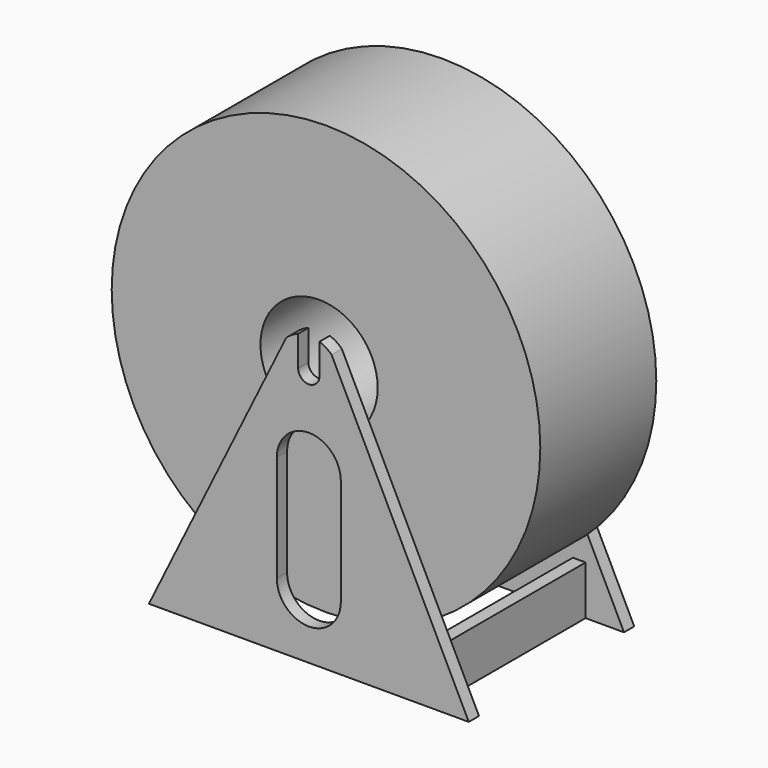
from build123d import *

# Parameters (mm, degrees)
F0_R      = 100.5
F0_R_2    = 27.5
F1_DEPTH  = 34
F3_DEPTH  = 6
F4_W      = 150
F4_H      = 6
F5_DEPTH  = 85
F9_DEPTH  = 122
F12_W     = 85
F12_H     = 36.2278819084
F13_DEPTH = 172
F14_W     = 6
F14_H     = 23
F15_DEPTH = 85


# Not quite as in the source:
# - a feature of the source that left no trace in its solid (it failed there, or was rolled back) is left out
# - a feature names something its author has since deleted; it is built from what else it names


with BuildPart() as f1:
    # F0 (on Front) → F1 (new body, symmetric)
    with BuildSketch(Plane.XZ):
        with Locations((3.2501332462, 0)):
            Circle(F0_R)
        Circle(F0_R_2, mode=Mode.SUBTRACT)
    extrude(amount=F1_DEPTH, both=True)


with BuildPart() as f3:
    # F2 (on face) → F3 (new body)
    with BuildSketch(Plane.XZ.offset(34)):
        with BuildLine():
            ThreePointArc((82.7773839779, -61.4464514114), (0.9255990786, -100.4731135225), (-79.0337407783, -57.7028082117))
            Line((-79.0337407783, -57.7028082117), (-141.3309325666, -120))
            Line((-141.3309325666, -120), (141.3309325666, -120))
            Line((141.3309325666, -120), (82.7773839779, -61.4464514114))
        make_face()
        with BuildLine():
            ThreePointArc((26.9250120629, -5.5940794963), (0, -27.5), (-26.9250120629, -5.5940794963))
            Line((-26.9250120629, -5.5940794963), (-79.0337407783, -57.7028082117))
            ThreePointArc((-79.0337407783, -57.7028082117), (0.9255990786, -100.4731135225), (82.7773839779, -61.4464514114))
            Line((82.7773839779, -61.4464514114), (26.9250120629, -5.5940794963))
        make_face()
        with BuildLine():
            Line((-5, 0), (-5, 14.2304020351))
            ThreePointArc((-5, 14.2304020351), (-8.0329882483, 12.7661835285), (-10.6654662833, 10.6654662833))
            Line((-10.6654662833, 10.6654662833), (-26.9250120629, -5.5940794963))
            ThreePointArc((-26.9250120629, -5.5940794963), (0, -27.5), (26.9250120629, -5.5940794963))
            Line((26.9250120629, -5.5940794963), (10.6654662833, 10.6654662833))
            ThreePointArc((10.6654662833, 10.6654662833), (8.0329882483, 12.7661835285), (5, 14.2304020351))
            Line((5, 14.2304020351), (5, 0))
            ThreePointArc((5, 0), (0, -5), (-5, 0))
        make_face()
    extrude(amount=F3_DEPTH)

    # F4 (on face) → F5 (join)
    with BuildSketch(Plane(origin=(0, -34, 0), x_dir=(-1, 0, 0), z_dir=(0, 1, 0))):
        with Locations((0, -117)):
            Rectangle(F4_W, F4_H)
    extrude(amount=F5_DEPTH)

    # F7: F3 across plane


with BuildPart() as f3_1:
    add(f3.part)
    add(f3.part.mirror(Plane(origin=(0, 8.5, -94.3962931942), x_dir=(-1, 0, 0), z_dir=(0, 1, 0))))

    # F8 (on face) → F9 (cut)
    with BuildSketch(Plane.XZ.offset(40)):
        Polygon((-141.3309325666, -120), (-75, -120), (-75, -54.6672668584), (-75, -53.6690674334), align=None)
        Polygon((75, -53.6690674334), (75, -120), (141.3309325666, -120), align=None)
        with BuildLine():
            Line((15, -90), (15, -40))
            ThreePointArc((15, -40), (0, -25), (-15, -40))
            Line((-15, -40), (-15, -90))
            ThreePointArc((-15, -90), (0, -105), (15, -90))
        make_face()
        Polygon((-75, -54.6672668584), (-75, -120), (-10.6654662833, 10.6654662833), (-75, -53.6690674334), align=None)
        Polygon((10.6654662833, 10.6654662833), (75, -120), (75, -53.6690674334), align=None)
    extrude(amount=-F9_DEPTH, mode=Mode.SUBTRACT)

    # F12 (on Right) → F13 (cut, symmetric)
    with BuildSketch(Plane.YZ):
        with Locations((8.5, -122.3534047604)):
            Rectangle(F12_W, F12_H)
    extrude(amount=F13_DEPTH, both=True, mode=Mode.SUBTRACT)

    # F14 (on face) → F15 (join, through all)
    with BuildSketch(Plane(origin=(0, -34, 0), x_dir=(-1, 0, 0), z_dir=(0, 1, 0))):
        with Locations((-54, -108.5)):
            Rectangle(F14_W, F14_H)
        with Locations((54, -108.5)):
            Rectangle(F14_W, F14_H)
    extrude(amount=F15_DEPTH)


solid = Compound([f1.part, f3_1.part])
